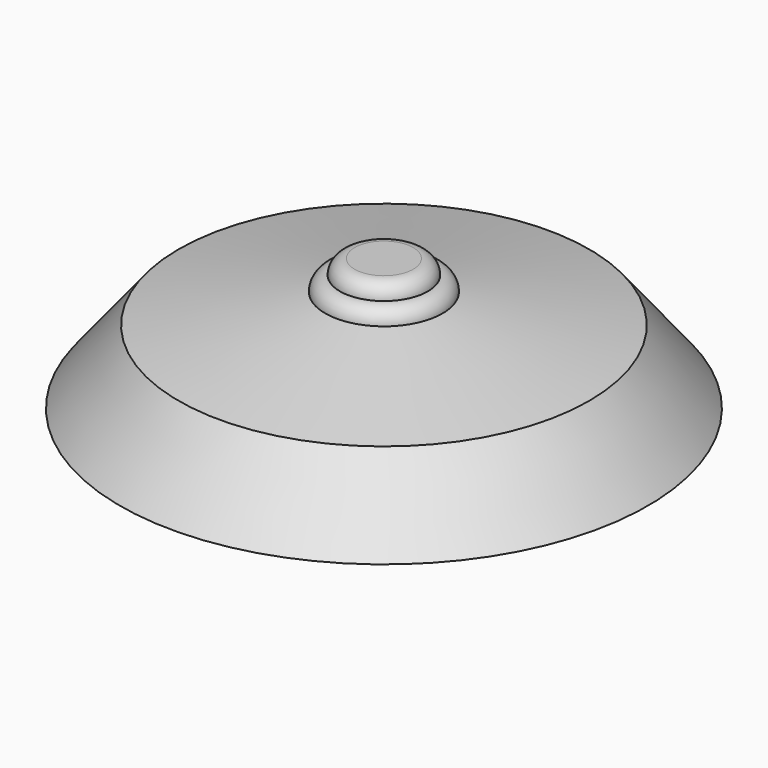
from build123d import *

# Parameters (mm, degrees)
F2_R = 4.99999


# Not quite as in the source:
# - a fillet or chamfer is up to 0.001 mm smaller than in the source, because OpenCascade refuses the exact size


with BuildPart() as f1:
    # F0 (on Front) → F1 (revolve)
    with BuildSketch(Plane.XZ):
        Polygon((-70, 25), (-90, 0), (0, 0), (0, 45), (-15, 45), (-15, 40), (-20, 40), (-20, 35), align=None)
    revolve(axis=Axis((0, 0, 22.5), (0, 0, -1)))

    # F2 (radius 5 in the source; OpenCascade refuses exactly that, so slightly less here)
    f2_edges = [f1.edges().sort_by_distance(p)[0] for p in [
        (20, 0, 40),
        (15, 0, 45),
    ]]
    fillet(f2_edges, radius=F2_R)


solid = f1.part
